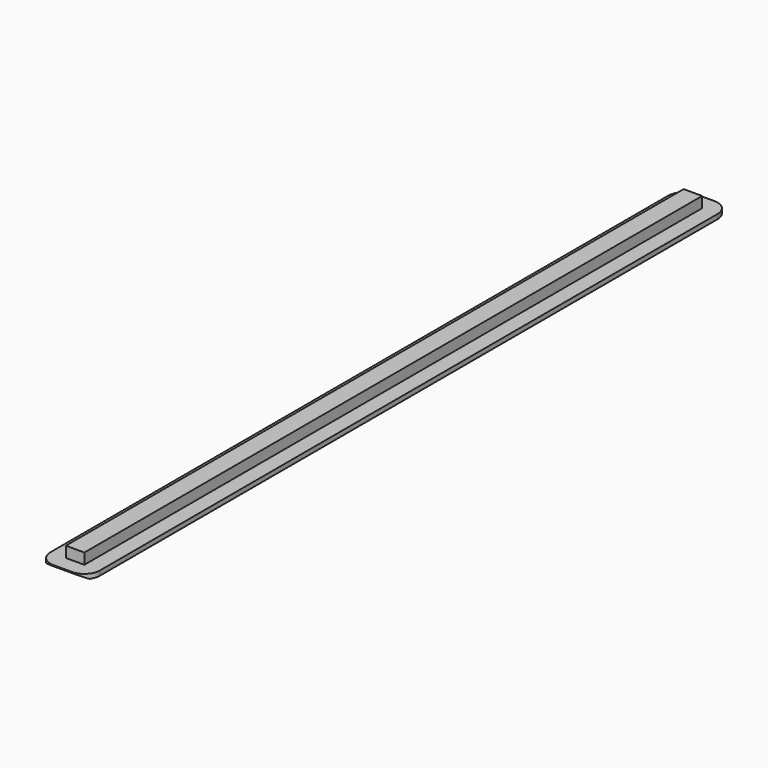
from build123d import *

# Parameters (mm, degrees)
F0_W        = 6.4
F0_H        = 104
F0_W_2      = 2.4
F0_H_2      = 100
F1_DEPTH    = 0.6
F2_DEPTH    = 2
F3_R        = 2
F4_T1_DEPTH = 6.5393372074


# Not quite as in the source:
# - a fillet or chamfer that OpenCascade refuses, or shapes differently, is made with other operations: its cross-section is extruded or revolved along the edge and cut away or added


with BuildPart() as f1:
    # F0 (on Top) → F1 (new body)
    with BuildSketch(Plane.XY):
        Rectangle(F0_W, F0_H)
        Rectangle(F0_W_2, F0_H_2, mode=Mode.SUBTRACT)
    extrude(amount=F1_DEPTH)

    # F0 (on Top) → F2 (join)
    with BuildSketch(Plane.XY):
        Rectangle(F0_W_2, F0_H_2)
    extrude(amount=F2_DEPTH)

    # F3
    f3_edges = [f1.edges().sort_by_distance(p)[0] for p in [
        (-3.2, -52, 0.3),
        (-3.2, 52, 0.3),
        (3.2, 52, 0.3),
        (3.2, -52, 0.3),
    ]]
    fillet(f3_edges, radius=F3_R)

    # F4: chamfer of 0.8 x 0.4618802154 on 1 edges, made by hand

    # F4_s2 → F4_t1 (cut)
    with BuildSketch(Plane.YZ.offset(-3.2696686037)):
        Polygon((-51.2, 0), (-52, 0.4618802154), (-52, 0), align=None)
    extrude(amount=F4_T1_DEPTH, mode=Mode.SUBTRACT)


solid = f1.part
